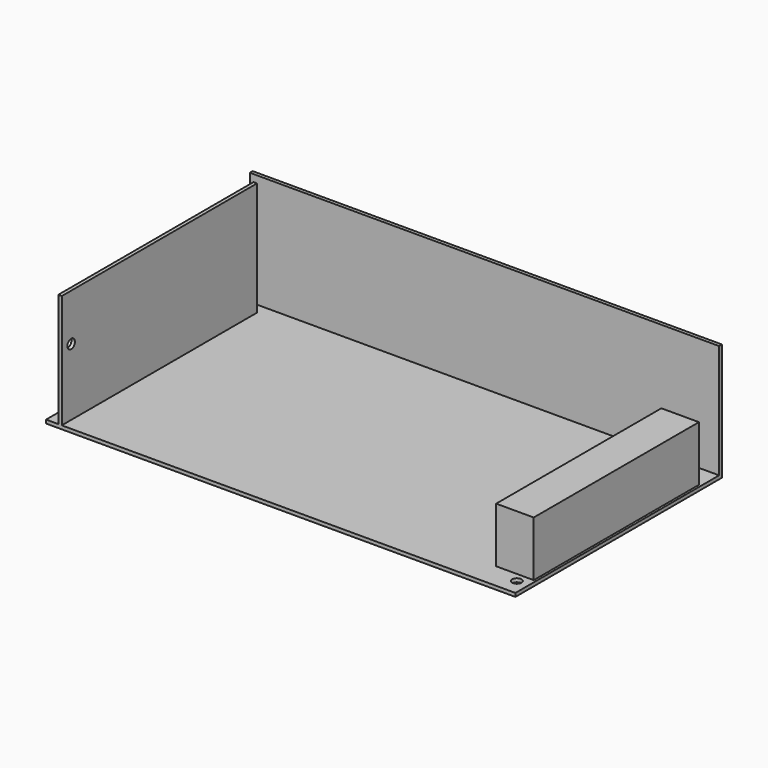
from build123d import *

# Parameters (mm, degrees)
F0_R     = 2
F0_W     = 16
F0_H     = 88
F2_DEPTH = 1.5
F0_W_2   = 1.5
F0_H_2   = 104
F3_DEPTH = 50
F4_DEPTH = 25
F5_D     = 4


# Not quite as in the source:
# - the program builds the solid bodies; features that only make, move or delete a surface that nothing else refers to are left out


with BuildPart() as f2:
    # F0 (on Top) → F2 (new body)
    with BuildSketch(Plane.XY):
        Polygon((100, 53.5), (-100, 53.5), (-100, -55), (-94.811744988, -55), (-94.811744988, 49), (-93.311744988, 49), (-93.311744988, -55), (100, -55), align=None)
        with Locations((95, -48)):
            Circle(F0_R, mode=Mode.SUBTRACT)
        with Locations((91, 0)):
            Rectangle(F0_W, F0_H, mode=Mode.SUBTRACT)
        with Locations((91, 0)):
            Rectangle(F0_W, F0_H)
    extrude(amount=F2_DEPTH)

    # F0 (on Top) → F3 (join)
    with BuildSketch(Plane.XY):
        Polygon((-58.6367584765, 55), (-100, 55), (-100, 53.5), (100, 53.5), (100, 55), (72.2615793347, 55), align=None)
        with Locations((-94.061744988, -3)):
            Rectangle(F0_W_2, F0_H_2)
    extrude(amount=F3_DEPTH)

    # F0 (on Top) → F4 (join)
    with BuildSketch(Plane.XY):
        with Locations((91, 0)):
            Rectangle(F0_W, F0_H)
    extrude(amount=F4_DEPTH)

    # F5 (through all)
    with Locations(Plane.YZ):
        with Locations((-50, 30)):
            Hole(F5_D / 2)


solid = f2.part
